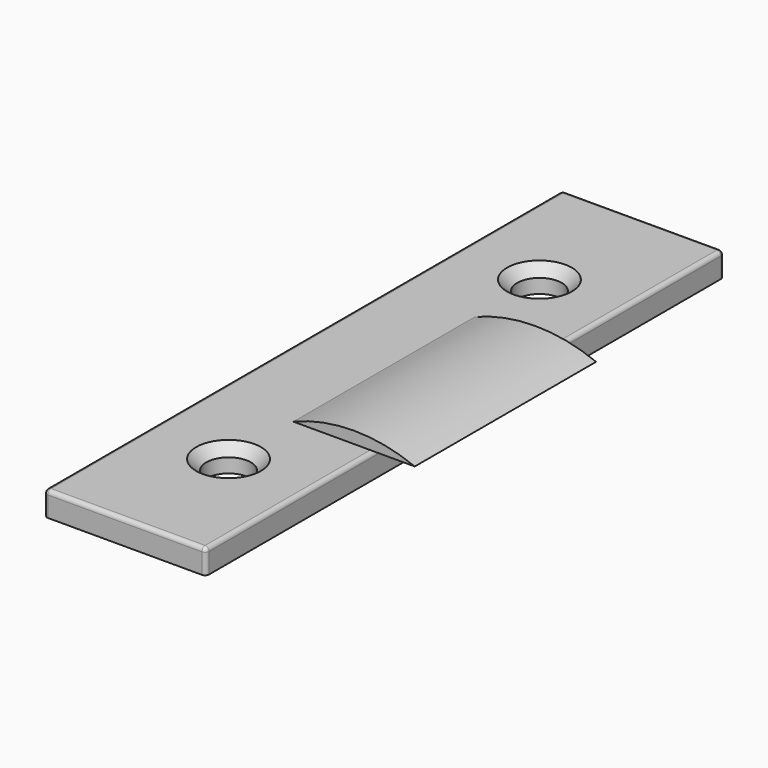
from build123d import *

# Parameters (mm, degrees)
F0_W           = 20
F0_H           = 80
F1_DEPTH       = 3
F5_D           = 5.5
F5_DEPTH       = 15
F5_CSINK_D     = 8
F5_CSINK_ANGLE = 90
F5_TIP         = 1.6523667023
F7_R           = 0.5
F10_DEPTH      = 28


# Not quite as in the source:
# - two fillets or chamfers of one size are made in one step


with BuildPart() as f1:
    # F0 (on Top) → F1 (new body)
    with BuildSketch(Plane.XY):
        with Locations((0, 24)):
            Rectangle(F0_W, F0_H)
    extrude(amount=F1_DEPTH)

    # F5
    with Locations(Plane.XY.offset(3)):
        with Locations((0, 0), (0, 48)):
            CounterSinkHole(F5_D / 2, F5_CSINK_D / 2, depth=F5_DEPTH, counter_sink_angle=F5_CSINK_ANGLE)
            with Locations((0, 0, -(F5_DEPTH + F5_TIP / 2))):  # 118° drill point
                Cone(0, F5_D / 2, F5_TIP, mode=Mode.SUBTRACT)

    # F7
    f7_edges = [f1.edges().sort_by_distance(p)[0] for p in [
        (0, 64, 3),
        (-10, 24, 3),
        (10, 24, 3),
        (-10, -16, 1.5),
        (-10, 64, 1.5),
        (10, 64, 1.5),
        (10, -16, 1.5),
        (0, -16, 3),
    ]]
    fillet(f7_edges, radius=F7_R)

    # F9 (on offset) → F10 (join)
    with BuildSketch(Plane.XZ.offset(-10)):
        with BuildLine():
            ThreePointArc((13, 3), (7.5, 3.860863499), (2, 3))
            Line((2, 3), (10, 3))
            Line((10, 3), (13, 3))
        make_face()
        with BuildLine():
            Line((0, 3), (2, 3))
            ThreePointArc((2, 3), (7.5, 3.860863499), (13, 3))
            Line((13, 3), (15, 3))
            ThreePointArc((15, 3), (7.5, 4.4595037823), (0, 3))
        make_face()
    extrude(amount=-F10_DEPTH)


solid = f1.part
